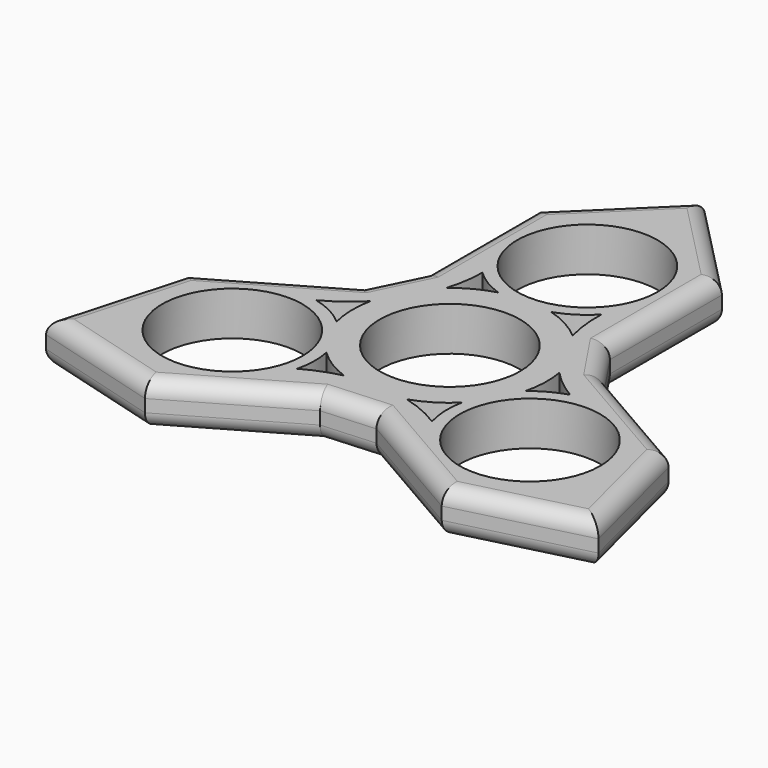
from build123d import *

# Parameters (mm, degrees)
F0_R     = 11.2
F1_DEPTH = 7
F3_DEPTH = 7
F4_DEPTH = 7
F5_R     = 2.5


# Not quite as in the source:
# - the program builds the solid bodies; features that only make, move or delete a surface that nothing else refers to are left out


with BuildPart() as f1:
    # F0 (on Top) → F1 (new body)
    with BuildSketch(Plane.XY):
        Polygon((-15.1401171461, 36.1142084002), (-15.1401171461, 14.037729241), (-18.916093286, 6.3695226165), (-38.2596134255, -4.7984639431), (-44.0662825692, -25.4416801035), (-23.7057633391, -31.1688302649), (-4.5869715611, -20.1305906853), (3.9418782472, -19.5665786343), (23.2853983866, -30.7345651939), (44.0662825692, -25.4416801035), (38.8458804852, -4.9453781354), (19.7270887072, 6.0928614443), (14.9742150389, 13.1970560178), (14.9742150389, 35.533029137), (0, 50.8833602071), align=None)
        with Locations((-23.7459174679, -13.7097118422)):
            Circle(F0_R, mode=Mode.SUBTRACT)
        with BuildLine():
            ThreePointArc((-5.2235825218, -14.5932924879), (-8.1486251459, -15.4948890799), (-10.9142807021, -16.8063387022))
            ThreePointArc((-10.9142807021, -16.8063387022), (-10.5484153212, -13.966494024), (-10.8035365954, -11.1145668846))
            ThreePointArc((-10.8035365954, -11.1145668846), (-8.2001536422, -13.1532307911), (-5.2235825218, -14.5932924879))
        make_face(mode=Mode.SUBTRACT)
        with BuildLine():
            ThreePointArc((-15.1785458421, 3.1403417202), (-15.4963179195, -0.3378327056), (-15.0272655718, -3.7988537))
            ThreePointArc((-15.0272655718, -3.7988537), (-17.6493915658, -2.0019207643), (-20.6250668218, -0.88394515))
            ThreePointArc((-20.6250668218, -0.88394515), (-17.7408860989, 0.9104067971), (-15.1785458421, 3.1403417202))
        make_face(mode=Mode.SUBTRACT)
        with BuildLine():
            ThreePointArc((4.8696572148, -14.7151771518), (8.040730665, -13.2512886306), (10.8035365954, -11.1145668846))
            ThreePointArc((10.8035365954, -11.1145668846), (10.5584100211, -14.2838610751), (11.0780523663, -17.4198592474))
            ThreePointArc((11.0780523663, -17.4198592474), (8.0820076354, -15.8192614458), (4.8696572148, -14.7151771518))
        make_face(mode=Mode.SUBTRACT)
        with Locations((23.7459174679, -13.7097118422)):
            Circle(F0_R, mode=Mode.SUBTRACT)
        with BuildLine():
            ThreePointArc((15.2499532803, 2.7728910813), (17.493280145, 0.6905281577), (20.0118566117, -1.0488750009))
            ThreePointArc((20.0118566117, -1.0488750009), (17.3695462872, -2.1519486258), (15.0272655718, -3.7988537))
            ThreePointArc((15.0272655718, -3.7988537), (15.491108828, -0.5249259735), (15.2499532803, 2.7728910813))
        make_face(mode=Mode.SUBTRACT)
        Circle(F0_R, mode=Mode.SUBTRACT)
        with BuildLine():
            ThreePointArc((-9.0975759097, 17.8552137031), (-6.821130966, 16.1184426499), (-4.2237289764, 14.9134205846))
            ThreePointArc((-4.2237289764, 14.9134205846), (-7.2909551859, 13.6781567646), (-10.0263707585, 11.8204014066))
            ThreePointArc((-10.0263707585, 11.8204014066), (-9.3446549991, 14.8043609222), (-9.0975759097, 17.8552137031))
        make_face(mode=Mode.SUBTRACT)
        with BuildLine():
            ThreePointArc((4.2237289764, 14.9134205846), (7.0909815446, 16.2857818394), (9.5470144555, 18.3038043974))
            ThreePointArc((9.5470144555, 18.3038043974), (9.6588784635, 14.9088546487), (10.3088886273, 11.5748354317))
            ThreePointArc((10.3088886273, 11.5748354317), (7.4555872545, 13.5891213362), (4.2237289764, 14.9134205846))
        make_face(mode=Mode.SUBTRACT)
        with Locations((0, 27.4194236845)):
            Circle(F0_R, mode=Mode.SUBTRACT)
    extrude(amount=F1_DEPTH)

    # F0 (on Top) → F3 (join)
    with BuildSketch(Plane.XY):
        Polygon((-15.1401171461, 36.1142084002), (-15.1401171461, 14.037729241), (-18.916093286, 6.3695226165), (-38.2596134255, -4.7984639431), (-44.0662825692, -25.4416801035), (-23.7057633391, -31.1688302649), (-4.5869715611, -20.1305906853), (3.9418782472, -19.5665786343), (23.2853983866, -30.7345651939), (44.0662825692, -25.4416801035), (38.8458804852, -4.9453781354), (19.7270887072, 6.0928614443), (14.9742150389, 13.1970560178), (14.9742150389, 35.533029137), (0, 50.8833602071), align=None)
        with Locations((-23.7459174679, -13.7097118422)):
            Circle(F0_R, mode=Mode.SUBTRACT)
        with BuildLine():
            ThreePointArc((-5.2235825218, -14.5932924879), (-8.1486251459, -15.4948890799), (-10.9142807021, -16.8063387022))
            ThreePointArc((-10.9142807021, -16.8063387022), (-10.5484153212, -13.966494024), (-10.8035365954, -11.1145668846))
            ThreePointArc((-10.8035365954, -11.1145668846), (-8.2001536422, -13.1532307911), (-5.2235825218, -14.5932924879))
        make_face(mode=Mode.SUBTRACT)
        with BuildLine():
            ThreePointArc((-15.1785458421, 3.1403417202), (-15.4963179195, -0.3378327056), (-15.0272655718, -3.7988537))
            ThreePointArc((-15.0272655718, -3.7988537), (-17.6493915658, -2.0019207643), (-20.6250668218, -0.88394515))
            ThreePointArc((-20.6250668218, -0.88394515), (-17.7408860989, 0.9104067971), (-15.1785458421, 3.1403417202))
        make_face(mode=Mode.SUBTRACT)
        with BuildLine():
            ThreePointArc((4.8696572148, -14.7151771518), (8.040730665, -13.2512886306), (10.8035365954, -11.1145668846))
            ThreePointArc((10.8035365954, -11.1145668846), (10.5584100211, -14.2838610751), (11.0780523663, -17.4198592474))
            ThreePointArc((11.0780523663, -17.4198592474), (8.0820076354, -15.8192614458), (4.8696572148, -14.7151771518))
        make_face(mode=Mode.SUBTRACT)
        with Locations((23.7459174679, -13.7097118422)):
            Circle(F0_R, mode=Mode.SUBTRACT)
        with BuildLine():
            ThreePointArc((15.2499532803, 2.7728910813), (17.493280145, 0.6905281577), (20.0118566117, -1.0488750009))
            ThreePointArc((20.0118566117, -1.0488750009), (17.3695462872, -2.1519486258), (15.0272655718, -3.7988537))
            ThreePointArc((15.0272655718, -3.7988537), (15.491108828, -0.5249259735), (15.2499532803, 2.7728910813))
        make_face(mode=Mode.SUBTRACT)
        Circle(F0_R, mode=Mode.SUBTRACT)
        with BuildLine():
            ThreePointArc((-9.0975759097, 17.8552137031), (-6.821130966, 16.1184426499), (-4.2237289764, 14.9134205846))
            ThreePointArc((-4.2237289764, 14.9134205846), (-7.2909551859, 13.6781567646), (-10.0263707585, 11.8204014066))
            ThreePointArc((-10.0263707585, 11.8204014066), (-9.3446549991, 14.8043609222), (-9.0975759097, 17.8552137031))
        make_face(mode=Mode.SUBTRACT)
        with BuildLine():
            ThreePointArc((4.2237289764, 14.9134205846), (7.0909815446, 16.2857818394), (9.5470144555, 18.3038043974))
            ThreePointArc((9.5470144555, 18.3038043974), (9.6588784635, 14.9088546487), (10.3088886273, 11.5748354317))
            ThreePointArc((10.3088886273, 11.5748354317), (7.4555872545, 13.5891213362), (4.2237289764, 14.9134205846))
        make_face(mode=Mode.SUBTRACT)
        with Locations((0, 27.4194236845)):
            Circle(F0_R, mode=Mode.SUBTRACT)
    extrude(amount=F3_DEPTH)

    # F0 (on Top) → F4 (join)
    with BuildSketch(Plane.XY):
        Polygon((-15.1401171461, 36.1142084002), (-15.1401171461, 14.037729241), (-18.916093286, 6.3695226165), (-38.2596134255, -4.7984639431), (-44.0662825692, -25.4416801035), (-23.7057633391, -31.1688302649), (-4.5869715611, -20.1305906853), (3.9418782472, -19.5665786343), (23.2853983866, -30.7345651939), (44.0662825692, -25.4416801035), (38.8458804852, -4.9453781354), (19.7270887072, 6.0928614443), (14.9742150389, 13.1970560178), (14.9742150389, 35.533029137), (0, 50.8833602071), align=None)
        with Locations((-23.7459174679, -13.7097118422)):
            Circle(F0_R, mode=Mode.SUBTRACT)
        with BuildLine():
            ThreePointArc((-5.2235825218, -14.5932924879), (-8.1486251459, -15.4948890799), (-10.9142807021, -16.8063387022))
            ThreePointArc((-10.9142807021, -16.8063387022), (-10.5484153212, -13.966494024), (-10.8035365954, -11.1145668846))
            ThreePointArc((-10.8035365954, -11.1145668846), (-8.2001536422, -13.1532307911), (-5.2235825218, -14.5932924879))
        make_face(mode=Mode.SUBTRACT)
        with BuildLine():
            ThreePointArc((-15.1785458421, 3.1403417202), (-15.4963179195, -0.3378327056), (-15.0272655718, -3.7988537))
            ThreePointArc((-15.0272655718, -3.7988537), (-17.6493915658, -2.0019207643), (-20.6250668218, -0.88394515))
            ThreePointArc((-20.6250668218, -0.88394515), (-17.7408860989, 0.9104067971), (-15.1785458421, 3.1403417202))
        make_face(mode=Mode.SUBTRACT)
        with BuildLine():
            ThreePointArc((4.8696572148, -14.7151771518), (8.040730665, -13.2512886306), (10.8035365954, -11.1145668846))
            ThreePointArc((10.8035365954, -11.1145668846), (10.5584100211, -14.2838610751), (11.0780523663, -17.4198592474))
            ThreePointArc((11.0780523663, -17.4198592474), (8.0820076354, -15.8192614458), (4.8696572148, -14.7151771518))
        make_face(mode=Mode.SUBTRACT)
        with Locations((23.7459174679, -13.7097118422)):
            Circle(F0_R, mode=Mode.SUBTRACT)
        with BuildLine():
            ThreePointArc((15.2499532803, 2.7728910813), (17.493280145, 0.6905281577), (20.0118566117, -1.0488750009))
            ThreePointArc((20.0118566117, -1.0488750009), (17.3695462872, -2.1519486258), (15.0272655718, -3.7988537))
            ThreePointArc((15.0272655718, -3.7988537), (15.491108828, -0.5249259735), (15.2499532803, 2.7728910813))
        make_face(mode=Mode.SUBTRACT)
        Circle(F0_R, mode=Mode.SUBTRACT)
        with BuildLine():
            ThreePointArc((-9.0975759097, 17.8552137031), (-6.821130966, 16.1184426499), (-4.2237289764, 14.9134205846))
            ThreePointArc((-4.2237289764, 14.9134205846), (-7.2909551859, 13.6781567646), (-10.0263707585, 11.8204014066))
            ThreePointArc((-10.0263707585, 11.8204014066), (-9.3446549991, 14.8043609222), (-9.0975759097, 17.8552137031))
        make_face(mode=Mode.SUBTRACT)
        with BuildLine():
            ThreePointArc((4.2237289764, 14.9134205846), (7.0909815446, 16.2857818394), (9.5470144555, 18.3038043974))
            ThreePointArc((9.5470144555, 18.3038043974), (9.6588784635, 14.9088546487), (10.3088886273, 11.5748354317))
            ThreePointArc((10.3088886273, 11.5748354317), (7.4555872545, 13.5891213362), (4.2237289764, 14.9134205846))
        make_face(mode=Mode.SUBTRACT)
        with Locations((0, 27.4194236845)):
            Circle(F0_R, mode=Mode.SUBTRACT)
    extrude(amount=F4_DEPTH)

    # F5
    f5_edges = [f1.edges().sort_by_distance(p)[0] for p in [
        (-7.570059, 43.498784, 7),
        (-15.140117, 25.075969, 7),
        (-17.028105, 10.203626, 7),
        (-28.587853, 0.785529, 7),
        (-41.162948, -15.120072, 7),
        (-33.886023, -28.305255, 7),
        (-14.146367, -25.64971, 7),
        (-0.322547, -19.848585, 7),
        (13.613638, -25.150572, 7),
        (33.67584, -28.088123, 7),
        (41.456082, -15.193529, 7),
        (29.286485, 0.573742, 7),
        (17.350652, 9.644959, 7),
        (14.974215, 24.365043, 7),
        (7.487108, 43.208195, 7),
        (7.487108, 43.208195, 0),
        (-7.570059, 43.498784, 0),
        (-15.140117, 25.075969, 0),
        (-17.028105, 10.203626, 0),
        (-14.146367, -25.64971, 0),
        (-0.322547, -19.848585, 0),
        (13.613638, -25.150572, 0),
        (33.67584, -28.088123, 0),
        (41.456082, -15.193529, 0),
        (29.286485, 0.573742, 0),
        (17.350652, 9.644959, 0),
        (14.974215, 24.365043, 0),
        (-28.587853, 0.785529, 0),
        (-41.162948, -15.120072, 0),
        (-33.886023, -28.305255, 0),
    ]]
    fillet(f5_edges, radius=F5_R)


solid = f1.part
